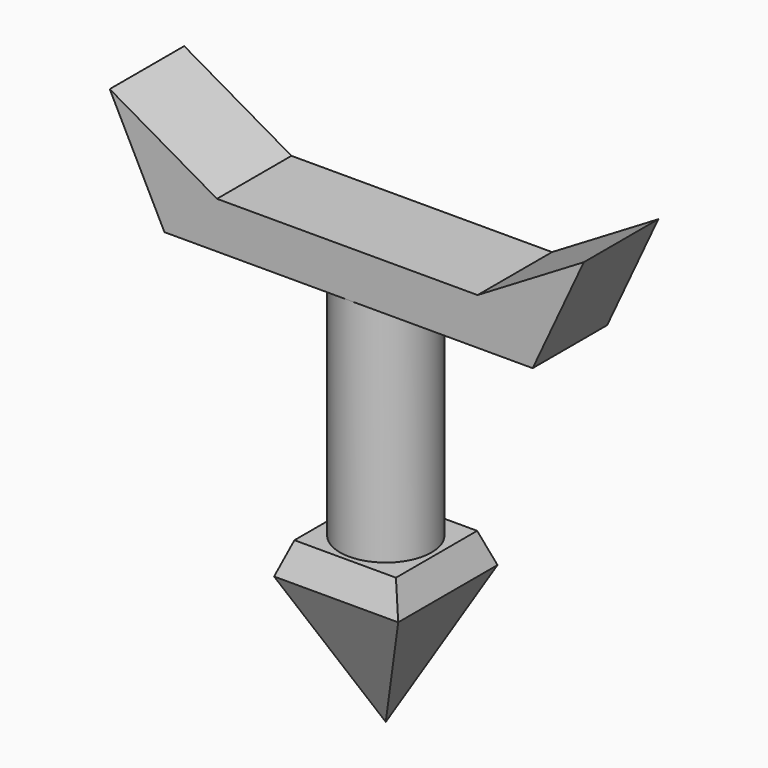
from build123d import *

# Parameters (mm, degrees)
F0_W      = 50.8
F0_H      = 50.8
F1_FACE_W = 50.8
F1_FACE_H = 50.8
F2_DEPTH  = 12.7
F2_TAPER  = 20
F3_R      = 18.7690091821
F4_DEPTH  = 101.6
F6_DEPTH  = 19.05


# Not quite as in the source:
# - an extrude whose draft closes it to a point is written as a loft to that point


with BuildPart() as f1:
    # F0 (on Top) → F1 section 0
    with BuildSketch(Plane.XY, mode=Mode.PRIVATE) as f1_s0:
        Rectangle(F0_W, F0_H)
    loft([f1_s0.sketch, Vertex(0, 0, -54.4704757809)], ruled=True)

    # F1_face (on face) → F2 (join)
    with BuildSketch(Plane.XY):
        Rectangle(F1_FACE_W, F1_FACE_H)
    extrude(amount=F2_DEPTH, taper=F2_TAPER)

    # F3 (on face) → F4 (join)
    with BuildSketch(Plane.XY.offset(12.7)):
        Circle(F3_R)
    extrude(amount=F4_DEPTH)

    # F5 (on Front) → F6 (join, symmetric)
    with BuildSketch(Plane.XZ):
        Polygon((96.2837857294, 150.2247155843), (52.8015196323, 124.2486089468), (-53.8494151779, 124.2486089468), (-97.7485626936, 149.513810873), (-75.3541216254, 105.235889554), (75.3541216254, 105.235889554), align=None)
    extrude(amount=F6_DEPTH, both=True)


solid = f1.part
